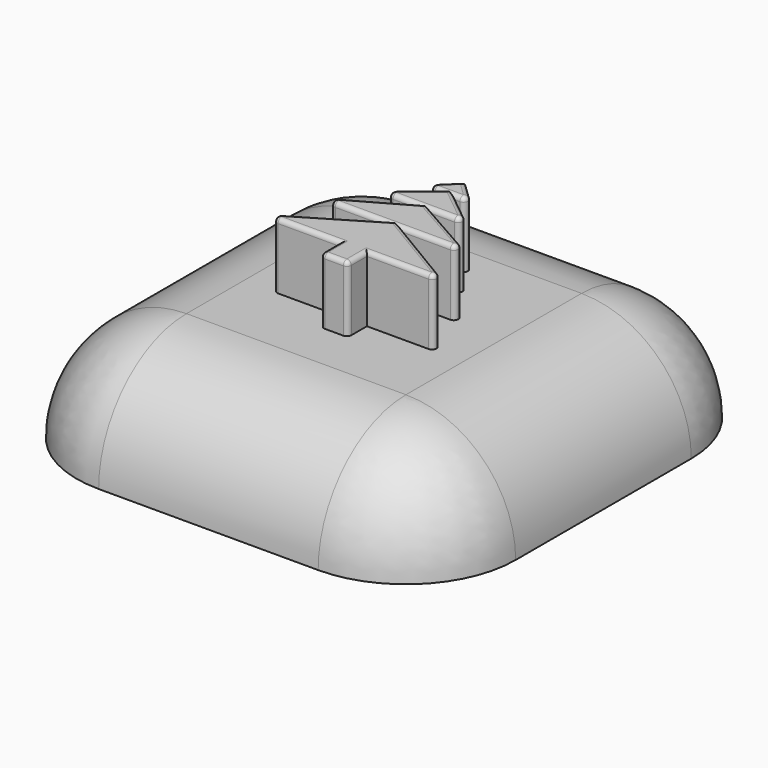
from build123d import *

# Parameters (mm, degrees)
F0_W          = 20
F0_H          = 20
F1_DEPTH      = 5
F2_R          = 4.99999
F3_T3_ANGLE   = 90
F3_T6_ANGLE   = 90
F3_T9_ANGLE   = 90
F3_T12_ANGLE  = 90
F3_T15_DEPTH  = 5
F3_T18_DEPTH  = 5
F3_T21_DEPTH  = 5
F3_T24_DEPTH  = 5
F5_DEPTH      = 3
F6_T1_DEPTH   = 4.0297756549
F6_T3_DEPTH   = 4.0297756549
F6_T5_DEPTH   = 2.2378753163
F6_T7_DEPTH   = 1.5910214623
F6_T9_DEPTH   = 2.4816952517
F6_T11_DEPTH  = 2.4816952517
F6_T16_DEPTH  = 2.7007100396
F6_T21_DEPTH  = 1.7701328723
F6_T26_DEPTH  = 1.7701328723
F6_T31_DEPTH  = 2.7007100396
F6_T36_DEPTH  = 3.9842649237
F6_T41_DEPTH  = 3.9842649237
F6_T46_DEPTH  = 5.3750440238
F6_T51_DEPTH  = 5.3750440238
F6_T56_DEPTH  = 4.5781609342
F6_T61_DEPTH  = 4.5781609342
F6_T66_DEPTH  = 3.1449194872
F6_T71_DEPTH  = 3.1449194872
F6_T77_DEPTH  = 2.7007100396
F6_T81_DEPTH  = 4.5781609342
F6_T88_DEPTH  = 1.7701328723
F6_T92_DEPTH  = 3.1449194872
F6_T99_DEPTH  = 3.1449194872
F6_T103_DEPTH = 1.7701328723
F6_T110_DEPTH = 2.7007100396
F6_T114_DEPTH = 4.5781609342
F6_T121_DEPTH = 5.3750440238
F6_T125_DEPTH = 3.9842649237
F6_T132_DEPTH = 3.9842649237
F6_T136_DEPTH = 5.3750440238
F6_T143_DEPTH = 4.5297756549
F6_T147_DEPTH = 2.0910214623
F6_T154_DEPTH = 2.0910214623
F6_T158_DEPTH = 4.5297756549
F7_T1_DEPTH   = 2.8
F7_T6_DEPTH   = 0.2
F7_T12_DEPTH  = 0.2
F7_T18_DEPTH  = 0.2
F7_T24_DEPTH  = 0.2
F7_S29_W      = 0.2
F7_S29_H      = 0.2
F7_T30_DEPTH  = 0.2
F7_S35_W      = 0.2
F7_S35_H      = 0.2
F7_T36_DEPTH  = 0.2
F7_T42_DEPTH  = 0.2
F7_T48_DEPTH  = 0.2
F7_T54_DEPTH  = 0.2
F7_T60_DEPTH  = 0.2


# Not quite as in the source:
# - a fillet or chamfer that OpenCascade refuses, or shapes differently, is made with other operations: its cross-section is extruded or revolved along the edge and cut away or added
# - a fillet or chamfer is up to 0.001 mm smaller than in the source, because OpenCascade refuses the exact size


with BuildPart() as f1:
    # F0 (on Top) → F1 (new body)
    with BuildSketch(Plane.XY):
        Rectangle(F0_W, F0_H)
    extrude(amount=-F1_DEPTH)

    # F2 (radius 5 in the source; OpenCascade refuses exactly that, so slightly less here)
    f2_edges = [f1.edges().sort_by_distance(p)[0] for p in [
        (0, 10, 0),
        (-10, 0, 0),
        (0, -10, 0),
        (10, 0, 0),
    ]]
    fillet(f2_edges, radius=F2_R)

    # F3: fillet of radius 5 on 5 edges, made by hand


with BuildPart() as f3_tool1:
    # F3_s2 → F3_t3 (revolve)
    with BuildSketch(Plane.YZ.offset(-5)):
        with BuildLine():
            ThreePointArc((5.00001, 0), (8.5355368349, -1.4644631651), (10, -4.99999))
            Line((10, -4.99999), (10, 0))
            Line((10, 0), (5.00001, 0))
        make_face()
    revolve(axis=Axis((-5, 5, 0), (0, 0, 1)), revolution_arc=F3_T3_ANGLE)


with BuildPart() as f3_tool4:
    # F3_s5 → F3_t6 (revolve)
    with BuildSketch(Plane.XZ.offset(-5)):
        with BuildLine():
            ThreePointArc((5.00001, 0), (8.5355368349, -1.4644631651), (10, -4.99999))
            Line((10, -4.99999), (10, 0))
            Line((10, 0), (5.00001, 0))
        make_face()
    revolve(axis=Axis((5, 5, 0), (0, 0, 1)), revolution_arc=F3_T6_ANGLE)


with BuildPart() as f3_tool7:
    # F3_s8 → F3_t9 (revolve)
    with BuildSketch(Plane.YZ.offset(5)):
        with BuildLine():
            ThreePointArc((-5.00001, 0), (-8.5355368349, -1.4644631651), (-10, -4.99999))
            Line((-10, -4.99999), (-10, 0))
            Line((-10, 0), (-5.00001, 0))
        make_face()
    revolve(axis=Axis((5, -5, 0), (0, 0, 1)), revolution_arc=F3_T9_ANGLE)


with BuildPart() as f3_tool10:
    # F3_s11 → F3_t12 (revolve)
    with BuildSketch(Plane.XZ.offset(5)):
        with BuildLine():
            ThreePointArc((-5.00001, 0), (-8.5355368349, -1.4644631651), (-10, -4.99999))
            Line((-10, -4.99999), (-10, 0))
            Line((-10, 0), (-5.00001, 0))
        make_face()
    revolve(axis=Axis((-5, -5, 0), (0, 0, 1)), revolution_arc=F3_T12_ANGLE)


with BuildPart() as f3_tool13:
    # F3_s14 → F3_t15 (new body)
    with BuildSketch(Plane.XY):
        with BuildLine():
            ThreePointArc((-5, -10), (-8.5355339059, -8.5355339059), (-10, -5))
            Line((-10, -5), (-10.1, -5))
            Line((-10.1, -5), (-10.1, -10.1))
            Line((-10.1, -10.1), (-5, -10.1))
            Line((-5, -10.1), (-5, -10))
        make_face()
    extrude(amount=-F3_T15_DEPTH)


with BuildPart() as f3_tool16:
    # F3_s17 → F3_t18 (new body)
    with BuildSketch(Plane.XY):
        with BuildLine():
            ThreePointArc((5, -10), (8.5355339059, -8.5355339059), (10, -5))
            Line((10, -5), (10.1, -5))
            Line((10.1, -5), (10.1, -10.1))
            Line((10.1, -10.1), (5, -10.1))
            Line((5, -10.1), (5, -10))
        make_face()
    extrude(amount=-F3_T18_DEPTH)


with BuildPart() as f3_tool19:
    # F3_s20 → F3_t21 (new body)
    with BuildSketch(Plane.XY):
        with BuildLine():
            ThreePointArc((10, 5), (8.5355339059, 8.5355339059), (5, 10))
            Line((5, 10), (5, 10.1))
            Line((5, 10.1), (10.1, 10.1))
            Line((10.1, 10.1), (10.1, 5))
            Line((10.1, 5), (10, 5))
        make_face()
    extrude(amount=-F3_T21_DEPTH)


with BuildPart() as f3_tool22:
    # F3_s23 → F3_t24 (new body)
    with BuildSketch(Plane.XY):
        with BuildLine():
            ThreePointArc((-10, 5), (-8.5355339059, 8.5355339059), (-5, 10))
            Line((-5, 10), (-5, 10.1))
            Line((-5, 10.1), (-10.1, 10.1))
            Line((-10.1, 10.1), (-10.1, 5))
            Line((-10.1, 5), (-10, 5))
        make_face()
    extrude(amount=-F3_T24_DEPTH)


with BuildPart() as f1_1:
    add(f1.part)

    # F3_t25: cut F3_tool1, F3_tool4, F3_tool7, F3_tool10, F3_tool13, F3_tool16, F3_tool19, F3_tool22
    add([f3_tool1.part, f3_tool4.part, f3_tool7.part, f3_tool10.part, f3_tool13.part, f3_tool16.part, f3_tool19.part, f3_tool22.part], mode=Mode.SUBTRACT)

    # F4 (on face) → F5 (join)
    with BuildSketch(Plane.XY):
        Polygon((1.0681818239, 3.6131960806), (0, 4.6400399879), (-1.0681818239, 3.6131960806), (-0.2980489517, 3.6131960806), (-1.9666701555, 2.2654635832), (-0.2659601159, 2.2654635832), (-3.3785805572, 0.5005755811), (-0.3943156335, 0.5005755811), (-4.148713313, -1.7456453061), (-0.6189376581, -1.7456453061), (-0.6189376581, -2.8366667684), (0, -2.8366667684), (0.6189376581, -2.8366667684), (0.6189376581, -1.7456453061), (4.148713313, -1.7456453061), (0.3943156335, 0.5005755811), (3.3785805572, 0.5005755811), (0.2659601159, 2.2654635832), (1.9666701555, 2.2654635832), (0.2980489517, 3.6131960806), align=None)
    extrude(amount=F5_DEPTH)

    # F6: fillet of radius 0.2 on 19 edges, made by hand

    # F6_s2 → F6_t1 (cut)
    with BuildSketch(Plane.YZ.offset(-4.648713313)):
        with BuildLine():
            ThreePointArc((-1.7456453061, 2.8), (-1.6870666623, 2.9414213562), (-1.5456453061, 3))
            Line((-1.5456453061, 3), (-1.7456453061, 3))
            Line((-1.7456453061, 3), (-1.7456453061, 2.8))
        make_face()
    extrude(amount=F6_T1_DEPTH, mode=Mode.SUBTRACT)

    # F6_s4 → F6_t3 (cut)
    with BuildSketch(Plane.YZ.offset(0.6189376581)):
        with BuildLine():
            ThreePointArc((-1.7456453061, 2.8), (-1.6870666623, 2.9414213562), (-1.5456453061, 3))
            Line((-1.5456453061, 3), (-1.7456453061, 3))
            Line((-1.7456453061, 3), (-1.7456453061, 2.8))
        make_face()
    extrude(amount=F6_T3_DEPTH, mode=Mode.SUBTRACT)

    # F6_s6 → F6_t5 (cut)
    with BuildSketch(Plane.YZ.offset(-1.1189376581)):
        with BuildLine():
            ThreePointArc((-2.8366667684, 2.8), (-2.7780881247, 2.9414213562), (-2.6366667684, 3))
            Line((-2.6366667684, 3), (-2.8366667684, 3))
            Line((-2.8366667684, 3), (-2.8366667684, 2.8))
        make_face()
    extrude(amount=F6_T5_DEPTH, mode=Mode.SUBTRACT)

    # F6_s8 → F6_t7 (cut)
    with BuildSketch(Plane.XZ.offset(1.7456453061)):
        with BuildLine():
            ThreePointArc((-0.6189376581, 2.8), (-0.5603590144, 2.9414213562), (-0.4189376581, 3))
            Line((-0.4189376581, 3), (-0.6189376581, 3))
            Line((-0.6189376581, 3), (-0.6189376581, 2.8))
        make_face()
        with BuildLine():
            ThreePointArc((0.6189376581, 2.8), (0.5603590144, 2.9414213562), (0.4189376581, 3))
            Line((0.4189376581, 3), (0.6189376581, 3))
            Line((0.6189376581, 3), (0.6189376581, 2.8))
        make_face()
    extrude(amount=F6_T7_DEPTH, mode=Mode.SUBTRACT)

    # F6_s10 → F6_t9 (cut)
    with BuildSketch(Plane(origin=(-0.8895730107, 0.8551471348, 0), x_dir=(0, 0, 1), z_dir=(-0.7209187063, 0.6930196382, 0))):
        with BuildLine():
            ThreePointArc((2.8, 3.345091625), (2.9414213562, 3.2865129813), (3, 3.145091625))
            Line((3, 3.145091625), (3, 3.345091625))
            Line((3, 3.345091625), (2.8, 3.345091625))
        make_face()
    extrude(amount=F6_T9_DEPTH, mode=Mode.SUBTRACT)

    # F6_s12 → F6_t11 (cut)
    with BuildSketch(Plane(origin=(2.6786735409, 2.5750106803, 0), x_dir=(0, 0, 1), z_dir=(-0.7209187063, -0.6930196382, 0))):
        with BuildLine():
            ThreePointArc((2.8, 3.345091625), (2.9414213562, 3.2865129813), (3, 3.145091625))
            Line((3, 3.145091625), (3, 3.345091625))
            Line((3, 3.345091625), (2.8, 3.345091625))
        make_face()
    extrude(amount=F6_T11_DEPTH, mode=Mode.SUBTRACT)


with BuildPart() as f6_tool14:
    # F6_s15 → F6_t16 (new body)
    with BuildSketch(Plane.YZ.offset(-2.4666701555)):
        with BuildLine():
            ThreePointArc((2.2654635832, 2.8), (2.3240422269, 2.9414213562), (2.4654635832, 3))
            Line((2.4654635832, 3), (2.2654635832, 3))
            Line((2.2654635832, 3), (2.2654635832, 2.8))
        make_face()
    extrude(amount=F6_T16_DEPTH)

    split(bisect_by=Plane(origin=(-1.036736214, 1.828425559, 0), x_dir=(0, 0, 1), z_dir=(-0.493238855, 0.8698939199, 0)), keep=Keep.TOP)


with BuildPart() as f1_2:
    add(f1_1.part)

    # F6_t13: cut F6_tool14
    add(f6_tool14.part, mode=Mode.SUBTRACT)


with BuildPart() as f6_tool19:
    # F6_s20 → F6_t21 (new body)
    with BuildSketch(Plane.YZ.offset(-1.5681818239)):
        with BuildLine():
            ThreePointArc((3.6131960806, 2.8), (3.6717747243, 2.9414213562), (3.8131960806, 3))
            Line((3.8131960806, 3), (3.6131960806, 3))
            Line((3.6131960806, 3), (3.6131960806, 2.8))
        make_face()
    extrude(amount=F6_T21_DEPTH)

    split(bisect_by=Plane(origin=(-1.8838358478, 2.3323682157, 0), x_dir=(0, 0, 1), z_dir=(-0.6283371033, 0.7779411833, 0)), keep=Keep.TOP)


with BuildPart() as f1_3:
    add(f1_2.part)

    # F6_t18: cut F6_tool19
    add(f6_tool19.part, mode=Mode.SUBTRACT)


with BuildPart() as f6_tool24:
    # F6_s25 → F6_t26 (new body)
    with BuildSketch(Plane.YZ.offset(-0.2019510483)):
        with BuildLine():
            ThreePointArc((3.6131960806, 2.8), (3.6717747243, 2.9414213562), (3.8131960806, 3))
            Line((3.8131960806, 3), (3.6131960806, 3))
            Line((3.6131960806, 3), (3.6131960806, 2.8))
        make_face()
    extrude(amount=F6_T26_DEPTH)

    split(bisect_by=Plane(origin=(1.8838358478, 2.3323682157, 0), x_dir=(0, 0, 1), z_dir=(0.6283371033, 0.7779411833, 0)), keep=Keep.TOP)


with BuildPart() as f1_4:
    add(f1_3.part)

    # F6_t23: cut F6_tool24
    add(f6_tool24.part, mode=Mode.SUBTRACT)


with BuildPart() as f6_tool29:
    # F6_s30 → F6_t31 (new body)
    with BuildSketch(Plane.YZ.offset(-0.2340398841)):
        with BuildLine():
            ThreePointArc((2.2654635832, 2.8), (2.3240422269, 2.9414213562), (2.4654635832, 3))
            Line((2.4654635832, 3), (2.2654635832, 3))
            Line((2.2654635832, 3), (2.2654635832, 2.8))
        make_face()
    extrude(amount=F6_T31_DEPTH)

    split(bisect_by=Plane(origin=(1.036736214, 1.828425559, 0), x_dir=(0, 0, 1), z_dir=(0.493238855, 0.8698939199, 0)), keep=Keep.TOP)


with BuildPart() as f1_5:
    add(f1_4.part)

    # F6_t28: cut F6_tool29
    add(f6_tool29.part, mode=Mode.SUBTRACT)


with BuildPart() as f6_tool34:
    # F6_s35 → F6_t36 (new body)
    with BuildSketch(Plane.YZ.offset(-0.1056843665)):
        with BuildLine():
            ThreePointArc((0.5005755811, 2.8), (0.5591542249, 2.9414213562), (0.7005755811, 3))
            Line((0.7005755811, 3), (0.5005755811, 3))
            Line((0.5005755811, 3), (0.5005755811, 2.8))
        make_face()
    extrude(amount=F6_T36_DEPTH)

    split(bisect_by=Plane(origin=(0.3244854875, 0.5423543019, 0), x_dir=(0, 0, 1), z_dir=(0.5134167508, 0.8581394059, 0)), keep=Keep.TOP)


with BuildPart() as f1_6:
    add(f1_5.part)

    # F6_t33: cut F6_tool34
    add(f6_tool34.part, mode=Mode.SUBTRACT)


with BuildPart() as f6_tool39:
    # F6_s40 → F6_t41 (new body)
    with BuildSketch(Plane.YZ.offset(-3.8785805572)):
        with BuildLine():
            ThreePointArc((0.5005755811, 2.8), (0.5591542249, 2.9414213562), (0.7005755811, 3))
            Line((0.7005755811, 3), (0.5005755811, 3))
            Line((0.5005755811, 3), (0.5005755811, 2.8))
        make_face()
    extrude(amount=F6_T41_DEPTH)

    split(bisect_by=Plane(origin=(-0.3244854875, 0.5423543019, 0), x_dir=(0, 0, 1), z_dir=(-0.5134167508, 0.8581394059, 0)), keep=Keep.TOP)


with BuildPart() as f1_7:
    add(f1_6.part)

    # F6_t38: cut F6_tool39
    add(f6_tool39.part, mode=Mode.SUBTRACT)


with BuildPart() as f6_tool44:
    # F6_s45 → F6_t46 (new body)
    with BuildSketch(Plane(origin=(4.2532975285, -2.5447079834, 0), x_dir=(0, 0, 1), z_dir=(-0.8581394059, 0.5134167508, 0))):
        with BuildLine():
            ThreePointArc((2.8, 0.6320118831), (2.9414213562, 0.5734332393), (3, 0.4320118831))
            Line((3, 0.4320118831), (3, 0.6320118831))
            Line((3, 0.6320118831), (2.8, 0.6320118831))
        make_face()
    extrude(amount=F6_T46_DEPTH)

    split(bisect_by=Plane.XZ.offset(-0.5005755811), keep=Keep.TOP)


with BuildPart() as f1_8:
    add(f1_7.part)

    # F6_t43: cut F6_tool44
    add(f6_tool44.part, mode=Mode.SUBTRACT)


with BuildPart() as f6_tool49:
    # F6_s50 → F6_t51 (new body)
    with BuildSketch(Plane(origin=(0.359239557, 0.2149296546, 0), x_dir=(0, 0, 1), z_dir=(-0.8581394059, -0.5134167508, 0))):
        with BuildLine():
            ThreePointArc((2.8, 0.6320118831), (2.9414213562, 0.5734332393), (3, 0.4320118831))
            Line((3, 0.4320118831), (3, 0.6320118831))
            Line((3, 0.6320118831), (2.8, 0.6320118831))
        make_face()
    extrude(amount=F6_T51_DEPTH)

    split(bisect_by=Plane.XZ.offset(-0.5005755811), keep=Keep.TOP)


with BuildPart() as f1_9:
    add(f1_8.part)

    # F6_t48: cut F6_tool49
    add(f6_tool49.part, mode=Mode.SUBTRACT)


with BuildPart() as f6_tool54:
    # F6_s55 → F6_t56 (new body)
    with BuildSketch(Plane(origin=(1.205723058, 0.6836574517, 0), x_dir=(0, 0, 1), z_dir=(-0.8698939199, -0.493238855, 0))):
        with BuildLine():
            ThreePointArc((2.8, 2.1018948599), (2.9414213562, 2.0433162161), (3, 1.9018948599))
            Line((3, 1.9018948599), (3, 2.1018948599))
            Line((3, 2.1018948599), (2.8, 2.1018948599))
        make_face()
    extrude(amount=F6_T56_DEPTH)

    split(bisect_by=Plane.XZ.offset(-2.2654635832), keep=Keep.TOP)


with BuildPart() as f1_10:
    add(f1_9.part)

    # F6_t53: cut F6_tool54
    add(f6_tool54.part, mode=Mode.SUBTRACT)


with BuildPart() as f6_tool59:
    # F6_s60 → F6_t61 (new body)
    with BuildSketch(Plane(origin=(2.7767913032, -1.5744694054, 0), x_dir=(0, 0, 1), z_dir=(-0.8698939199, 0.493238855, 0))):
        with BuildLine():
            ThreePointArc((2.8, 2.1018948599), (2.9414213562, 2.0433162161), (3, 1.9018948599))
            Line((3, 1.9018948599), (3, 2.1018948599))
            Line((3, 2.1018948599), (2.8, 2.1018948599))
        make_face()
    extrude(amount=F6_T61_DEPTH)

    split(bisect_by=Plane.XZ.offset(-2.2654635832), keep=Keep.TOP)


with BuildPart() as f1_11:
    add(f1_10.part)

    # F6_t58: cut F6_tool59
    add(f6_tool59.part, mode=Mode.SUBTRACT)


with BuildPart() as f6_tool64:
    # F6_s65 → F6_t66 (new body)
    with BuildSketch(Plane(origin=(0.4718048994, -0.3810731842, 0), x_dir=(0, 0, 1), z_dir=(-0.7779411833, 0.6283371033, 0))):
        with BuildLine():
            ThreePointArc((2.8, 2.9981292492), (2.9414213562, 2.9395506054), (3, 2.7981292492))
            Line((3, 2.7981292492), (3, 2.9981292492))
            Line((3, 2.9981292492), (2.8, 2.9981292492))
        make_face()
    extrude(amount=F6_T66_DEPTH)

    split(bisect_by=Plane.XZ.offset(-3.6131960806), keep=Keep.TOP)


with BuildPart() as f1_12:
    add(f1_11.part)

    # F6_t63: cut F6_tool64
    add(f6_tool64.part, mode=Mode.SUBTRACT)


with BuildPart() as f6_tool69:
    # F6_s70 → F6_t71 (new body)
    with BuildSketch(Plane(origin=(1.9747574877, 1.5949964165, 0), x_dir=(0, 0, 1), z_dir=(-0.7779411833, -0.6283371033, 0))):
        with BuildLine():
            ThreePointArc((2.8, 2.9981292492), (2.9414213562, 2.9395506054), (3, 2.7981292492))
            Line((3, 2.7981292492), (3, 2.9981292492))
            Line((3, 2.9981292492), (2.8, 2.9981292492))
        make_face()
    extrude(amount=F6_T71_DEPTH)

    split(bisect_by=Plane.XZ.offset(-3.6131960806), keep=Keep.TOP)


with BuildPart() as f1_13:
    add(f1_12.part)

    # F6_t68: cut F6_tool69
    add(f6_tool69.part, mode=Mode.SUBTRACT)


with BuildPart() as f6_tool75:
    # F6_s76 → F6_t77 (new body)
    with BuildSketch(Plane.YZ.offset(-2.4666701555)):
        with BuildLine():
            ThreePointArc((2.2654635832, 2.8), (2.3240422269, 2.9414213562), (2.4654635832, 3))
            Line((2.4654635832, 3), (2.2654635832, 3))
            Line((2.2654635832, 3), (2.2654635832, 2.8))
        make_face()
    extrude(amount=F6_T77_DEPTH)

    split(bisect_by=Plane(origin=(-1.036736214, 1.828425559, 0), x_dir=(0, 0, 1), z_dir=(0.493238855, -0.8698939199, 0)), keep=Keep.TOP)


with BuildPart() as f6_tool79:
    # F6_s80 → F6_t81 (new body)
    with BuildSketch(Plane(origin=(1.205723058, 0.6836574517, 0), x_dir=(0, 0, 1), z_dir=(-0.8698939199, -0.493238855, 0))):
        with BuildLine():
            ThreePointArc((2.8, 2.1018948599), (2.9414213562, 2.0433162161), (3, 1.9018948599))
            Line((3, 1.9018948599), (3, 2.1018948599))
            Line((3, 2.1018948599), (2.8, 2.1018948599))
        make_face()
    extrude(amount=F6_T81_DEPTH)

    split(bisect_by=Plane.XZ.offset(-2.2654635832), keep=Keep.BOTTOM)


with BuildPart() as f6_tool75_1:
    add(f6_tool75.part)

    # F6_t83: intersect F6_tool79
    add(f6_tool79.part, mode=Mode.INTERSECT)


with BuildPart() as f1_14:
    add(f1_13.part)

    # F6_t73: cut F6_tool75
    add(f6_tool75_1.part, mode=Mode.SUBTRACT)


with BuildPart() as f6_tool86:
    # F6_s87 → F6_t88 (new body)
    with BuildSketch(Plane.YZ.offset(-1.5681818239)):
        with BuildLine():
            ThreePointArc((3.6131960806, 2.8), (3.6717747243, 2.9414213562), (3.8131960806, 3))
            Line((3.8131960806, 3), (3.6131960806, 3))
            Line((3.6131960806, 3), (3.6131960806, 2.8))
        make_face()
    extrude(amount=F6_T88_DEPTH)

    split(bisect_by=Plane(origin=(-1.8838358478, 2.3323682157, 0), x_dir=(0, 0, 1), z_dir=(0.6283371033, -0.7779411833, 0)), keep=Keep.TOP)


with BuildPart() as f6_tool90:
    # F6_s91 → F6_t92 (new body)
    with BuildSketch(Plane(origin=(1.9747574877, 1.5949964165, 0), x_dir=(0, 0, 1), z_dir=(-0.7779411833, -0.6283371033, 0))):
        with BuildLine():
            ThreePointArc((2.8, 2.9981292492), (2.9414213562, 2.9395506054), (3, 2.7981292492))
            Line((3, 2.7981292492), (3, 2.9981292492))
            Line((3, 2.9981292492), (2.8, 2.9981292492))
        make_face()
    extrude(amount=F6_T92_DEPTH)

    split(bisect_by=Plane.XZ.offset(-3.6131960806), keep=Keep.BOTTOM)


with BuildPart() as f6_tool86_1:
    add(f6_tool86.part)

    # F6_t94: intersect F6_tool90
    add(f6_tool90.part, mode=Mode.INTERSECT)


with BuildPart() as f1_15:
    add(f1_14.part)

    # F6_t84: cut F6_tool86
    add(f6_tool86_1.part, mode=Mode.SUBTRACT)


with BuildPart() as f6_tool97:
    # F6_s98 → F6_t99 (new body)
    with BuildSketch(Plane(origin=(0.4718048994, -0.3810731842, 0), x_dir=(0, 0, 1), z_dir=(-0.7779411833, 0.6283371033, 0))):
        with BuildLine():
            ThreePointArc((2.8, 2.9981292492), (2.9414213562, 2.9395506054), (3, 2.7981292492))
            Line((3, 2.7981292492), (3, 2.9981292492))
            Line((3, 2.9981292492), (2.8, 2.9981292492))
        make_face()
    extrude(amount=F6_T99_DEPTH)

    split(bisect_by=Plane.XZ.offset(-3.6131960806), keep=Keep.BOTTOM)


with BuildPart() as f6_tool101:
    # F6_s102 → F6_t103 (new body)
    with BuildSketch(Plane.YZ.offset(-0.2019510483)):
        with BuildLine():
            ThreePointArc((3.6131960806, 2.8), (3.6717747243, 2.9414213562), (3.8131960806, 3))
            Line((3.8131960806, 3), (3.6131960806, 3))
            Line((3.6131960806, 3), (3.6131960806, 2.8))
        make_face()
    extrude(amount=F6_T103_DEPTH)

    split(bisect_by=Plane(origin=(1.8838358478, 2.3323682157, 0), x_dir=(0, 0, 1), z_dir=(-0.6283371033, -0.7779411833, 0)), keep=Keep.TOP)


with BuildPart() as f6_tool97_1:
    add(f6_tool97.part)

    # F6_t105: intersect F6_tool101
    add(f6_tool101.part, mode=Mode.INTERSECT)


with BuildPart() as f1_16:
    add(f1_15.part)

    # F6_t95: cut F6_tool97
    add(f6_tool97_1.part, mode=Mode.SUBTRACT)


with BuildPart() as f6_tool108:
    # F6_s109 → F6_t110 (new body)
    with BuildSketch(Plane.YZ.offset(-0.2340398841)):
        with BuildLine():
            ThreePointArc((2.2654635832, 2.8), (2.3240422269, 2.9414213562), (2.4654635832, 3))
            Line((2.4654635832, 3), (2.2654635832, 3))
            Line((2.2654635832, 3), (2.2654635832, 2.8))
        make_face()
    extrude(amount=F6_T110_DEPTH)

    split(bisect_by=Plane(origin=(1.036736214, 1.828425559, 0), x_dir=(0, 0, 1), z_dir=(-0.493238855, -0.8698939199, 0)), keep=Keep.TOP)


with BuildPart() as f6_tool112:
    # F6_s113 → F6_t114 (new body)
    with BuildSketch(Plane(origin=(2.7767913032, -1.5744694054, 0), x_dir=(0, 0, 1), z_dir=(-0.8698939199, 0.493238855, 0))):
        with BuildLine():
            ThreePointArc((2.8, 2.1018948599), (2.9414213562, 2.0433162161), (3, 1.9018948599))
            Line((3, 1.9018948599), (3, 2.1018948599))
            Line((3, 2.1018948599), (2.8, 2.1018948599))
        make_face()
    extrude(amount=F6_T114_DEPTH)

    split(bisect_by=Plane.XZ.offset(-2.2654635832), keep=Keep.BOTTOM)


with BuildPart() as f6_tool108_1:
    add(f6_tool108.part)

    # F6_t116: intersect F6_tool112
    add(f6_tool112.part, mode=Mode.INTERSECT)


with BuildPart() as f1_17:
    add(f1_16.part)

    # F6_t106: cut F6_tool108
    add(f6_tool108_1.part, mode=Mode.SUBTRACT)


with BuildPart() as f6_tool119:
    # F6_s120 → F6_t121 (new body)
    with BuildSketch(Plane(origin=(4.2532975285, -2.5447079834, 0), x_dir=(0, 0, 1), z_dir=(-0.8581394059, 0.5134167508, 0))):
        with BuildLine():
            ThreePointArc((2.8, 0.6320118831), (2.9414213562, 0.5734332393), (3, 0.4320118831))
            Line((3, 0.4320118831), (3, 0.6320118831))
            Line((3, 0.6320118831), (2.8, 0.6320118831))
        make_face()
    extrude(amount=F6_T121_DEPTH)

    split(bisect_by=Plane.XZ.offset(-0.5005755811), keep=Keep.BOTTOM)


with BuildPart() as f6_tool123:
    # F6_s124 → F6_t125 (new body)
    with BuildSketch(Plane.YZ.offset(-0.1056843665)):
        with BuildLine():
            ThreePointArc((0.5005755811, 2.8), (0.5591542249, 2.9414213562), (0.7005755811, 3))
            Line((0.7005755811, 3), (0.5005755811, 3))
            Line((0.5005755811, 3), (0.5005755811, 2.8))
        make_face()
    extrude(amount=F6_T125_DEPTH)

    split(bisect_by=Plane(origin=(0.3244854875, 0.5423543019, 0), x_dir=(0, 0, 1), z_dir=(-0.5134167508, -0.8581394059, 0)), keep=Keep.TOP)


with BuildPart() as f6_tool119_1:
    add(f6_tool119.part)

    # F6_t127: intersect F6_tool123
    add(f6_tool123.part, mode=Mode.INTERSECT)


with BuildPart() as f1_18:
    add(f1_17.part)

    # F6_t117: cut F6_tool119
    add(f6_tool119_1.part, mode=Mode.SUBTRACT)


with BuildPart() as f6_tool130:
    # F6_s131 → F6_t132 (new body)
    with BuildSketch(Plane.YZ.offset(-3.8785805572)):
        with BuildLine():
            ThreePointArc((0.5005755811, 2.8), (0.5591542249, 2.9414213562), (0.7005755811, 3))
            Line((0.7005755811, 3), (0.5005755811, 3))
            Line((0.5005755811, 3), (0.5005755811, 2.8))
        make_face()
    extrude(amount=F6_T132_DEPTH)

    split(bisect_by=Plane(origin=(-0.3244854875, 0.5423543019, 0), x_dir=(0, 0, 1), z_dir=(0.5134167508, -0.8581394059, 0)), keep=Keep.TOP)


with BuildPart() as f6_tool134:
    # F6_s135 → F6_t136 (new body)
    with BuildSketch(Plane(origin=(0.359239557, 0.2149296546, 0), x_dir=(0, 0, 1), z_dir=(-0.8581394059, -0.5134167508, 0))):
        with BuildLine():
            ThreePointArc((2.8, 0.6320118831), (2.9414213562, 0.5734332393), (3, 0.4320118831))
            Line((3, 0.4320118831), (3, 0.6320118831))
            Line((3, 0.6320118831), (2.8, 0.6320118831))
        make_face()
    extrude(amount=F6_T136_DEPTH)

    split(bisect_by=Plane.XZ.offset(-0.5005755811), keep=Keep.BOTTOM)


with BuildPart() as f6_tool130_1:
    add(f6_tool130.part)

    # F6_t138: intersect F6_tool134
    add(f6_tool134.part, mode=Mode.INTERSECT)


with BuildPart() as f1_19:
    add(f1_18.part)

    # F6_t128: cut F6_tool130
    add(f6_tool130_1.part, mode=Mode.SUBTRACT)


with BuildPart() as f6_tool141:
    # F6_s142 → F6_t143 (new body)
    with BuildSketch(Plane.YZ.offset(-4.648713313)):
        with BuildLine():
            ThreePointArc((-1.7456453061, 2.8), (-1.6870666623, 2.9414213562), (-1.5456453061, 3))
            Line((-1.5456453061, 3), (-1.7456453061, 3))
            Line((-1.7456453061, 3), (-1.7456453061, 2.8))
        make_face()
    extrude(amount=F6_T143_DEPTH)

    split(bisect_by=Plane.YZ.offset(-0.6189376581), keep=Keep.TOP)


with BuildPart() as f6_tool145:
    # F6_s146 → F6_t147 (new body)
    with BuildSketch(Plane.XZ.offset(1.2456453061)):
        with BuildLine():
            ThreePointArc((-0.6189376581, 2.8), (-0.5603590144, 2.9414213562), (-0.4189376581, 3))
            Line((-0.4189376581, 3), (-0.6189376581, 3))
            Line((-0.6189376581, 3), (-0.6189376581, 2.8))
        make_face()
    extrude(amount=F6_T147_DEPTH)

    split(bisect_by=Plane.XZ.offset(1.7456453061), keep=Keep.BOTTOM)


with BuildPart() as f6_tool141_1:
    add(f6_tool141.part)

    # F6_t149: intersect F6_tool145
    add(f6_tool145.part, mode=Mode.INTERSECT)


with BuildPart() as f1_20:
    add(f1_19.part)

    # F6_t139: cut F6_tool141
    add(f6_tool141_1.part, mode=Mode.SUBTRACT)


with BuildPart() as f6_tool152:
    # F6_s153 → F6_t154 (new body)
    with BuildSketch(Plane.XZ.offset(3.3366667684)):
        with BuildLine():
            ThreePointArc((0.6189376581, 2.8), (0.5603590144, 2.9414213562), (0.4189376581, 3))
            Line((0.4189376581, 3), (0.6189376581, 3))
            Line((0.6189376581, 3), (0.6189376581, 2.8))
        make_face()
    extrude(amount=-F6_T154_DEPTH)

    split(bisect_by=Plane.XZ.offset(1.7456453061), keep=Keep.BOTTOM)


with BuildPart() as f6_tool156:
    # F6_s157 → F6_t158 (new body)
    with BuildSketch(Plane.YZ.offset(0.1189376581)):
        with BuildLine():
            ThreePointArc((-1.7456453061, 2.8), (-1.6870666623, 2.9414213562), (-1.5456453061, 3))
            Line((-1.5456453061, 3), (-1.7456453061, 3))
            Line((-1.7456453061, 3), (-1.7456453061, 2.8))
        make_face()
    extrude(amount=F6_T158_DEPTH)

    split(bisect_by=Plane.YZ.offset(0.6189376581), keep=Keep.BOTTOM)


with BuildPart() as f6_tool152_1:
    add(f6_tool152.part)

    # F6_t160: intersect F6_tool156
    add(f6_tool156.part, mode=Mode.INTERSECT)


with BuildPart() as f1_21:
    add(f1_20.part)

    # F6_t150: cut F6_tool152
    add(f6_tool152_1.part, mode=Mode.SUBTRACT)

    # F7: fillet of radius 0.2 on 10 edges, made by hand

    # F7_s2 → F7_t1 (cut)
    with BuildSketch(Plane.XY):
        with BuildLine():
            ThreePointArc((0.7101421902, 3.9573798218), (0.7570601592, 3.738485801), (0.5715382625, 3.6131960806))
            Line((0.5715382625, 3.6131960806), (1.0681818239, 3.6131960806))
            Line((1.0681818239, 3.6131960806), (0.7101421902, 3.9573798218))
        make_face()
        with BuildLine():
            ThreePointArc((1.5264180486, 2.6210518198), (1.589321102, 2.3988214318), (1.400750628, 2.2654635832))
            Line((1.400750628, 2.2654635832), (1.9666701555, 2.2654635832))
            Line((1.9666701555, 2.2654635832), (1.5264180486, 2.6210518198))
        make_face()
        with BuildLine():
            ThreePointArc((2.7190180205, 0.8745543651), (2.8137555602, 0.6495645862), (2.6203702495, 0.5005755811))
            Line((2.6203702495, 0.5005755811), (3.3785805572, 0.5005755811))
            Line((3.3785805572, 0.5005755811), (2.7190180205, 0.8745543651))
        make_face()
        with BuildLine():
            ThreePointArc((3.5275638692, -1.3740174249), (3.6176570428, -1.598910791), (3.4248805191, -1.7456453061))
            Line((3.4248805191, -1.7456453061), (4.148713313, -1.7456453061))
            Line((4.148713313, -1.7456453061), (3.5275638692, -1.3740174249))
        make_face()
        with BuildLine():
            ThreePointArc((0.6189376581, -2.6366667684), (0.5603590144, -2.7780881247), (0.4189376581, -2.8366667684))
            Line((0.4189376581, -2.8366667684), (0.6189376581, -2.8366667684))
            Line((0.6189376581, -2.8366667684), (0.6189376581, -2.6366667684))
        make_face()
        with BuildLine():
            ThreePointArc((-0.4189376581, -2.8366667684), (-0.5603590144, -2.7780881247), (-0.6189376581, -2.6366667684))
            Line((-0.6189376581, -2.6366667684), (-0.6189376581, -2.8366667684))
            Line((-0.6189376581, -2.8366667684), (-0.4189376581, -2.8366667684))
        make_face()
        with BuildLine():
            ThreePointArc((-2.6203702495, 0.5005755811), (-2.8137555602, 0.6495645862), (-2.7190180205, 0.8745543651))
            Line((-2.7190180205, 0.8745543651), (-3.3785805572, 0.5005755811))
            Line((-3.3785805572, 0.5005755811), (-2.6203702495, 0.5005755811))
        make_face()
        with BuildLine():
            ThreePointArc((-1.400750628, 2.2654635832), (-1.589321102, 2.3988214318), (-1.5264180486, 2.6210518198))
            Line((-1.5264180486, 2.6210518198), (-1.9666701555, 2.2654635832))
            Line((-1.9666701555, 2.2654635832), (-1.400750628, 2.2654635832))
        make_face()
        with BuildLine():
            ThreePointArc((-0.5715382625, 3.6131960806), (-0.7570601592, 3.738485801), (-0.7101421902, 3.9573798218))
            Line((-0.7101421902, 3.9573798218), (-1.0681818239, 3.6131960806))
            Line((-1.0681818239, 3.6131960806), (-0.5715382625, 3.6131960806))
        make_face()
        with BuildLine():
            ThreePointArc((-3.4248805191, -1.7456453061), (-3.6176570428, -1.598910791), (-3.5275638692, -1.3740174249))
            Line((-3.5275638692, -1.3740174249), (-4.148713313, -1.7456453061))
            Line((-4.148713313, -1.7456453061), (-3.4248805191, -1.7456453061))
        make_face()
    extrude(amount=F7_T1_DEPTH, mode=Mode.SUBTRACT)


with BuildPart() as f7_tool4:
    # F7_s5 → F7_t6 (new body)
    with BuildSketch(Plane.XY.offset(2.8)):
        Polygon((-3.4248805191, -1.5456453061), (-3.4248805191, -1.7456453061), (-4.148713313, -1.7456453061), (-3.5275638692, -1.3740174249), align=None)
    extrude(amount=F7_T6_DEPTH)

    # F7_s7 → F7_t8 (revolve, cut)
    with BuildSketch(Plane(origin=(-3.4248805191, -1.5456453061, 2.8), x_dir=(0.9638826189, 0.2663274245, 0), z_dir=(0.2663274245, -0.9638826189, 0))):
        with BuildLine():
            ThreePointArc((0, -0.2), (0.2, 0), (0, 0.2))
            Line((0, 0.2), (0, -0.2))
        make_face()
    revolve(axis=Axis((-3.4248805191, -1.5456453061, 2.8), (0, 0, 1)), mode=Mode.SUBTRACT)


with BuildPart() as f1_22:
    add(f1_21.part)

    # F7_t3: cut F7_tool4
    add(f7_tool4.part, mode=Mode.SUBTRACT)


with BuildPart() as f7_tool10:
    # F7_s11 → F7_t12 (new body)
    with BuildSketch(Plane.XY.offset(2.8)):
        Polygon((-0.5715382625, 3.8131960806), (-0.5715382625, 3.6131960806), (-1.0681818239, 3.6131960806), (-0.7101421902, 3.9573798218), align=None)
    extrude(amount=F7_T12_DEPTH)

    # F7_s13 → F7_t14 (revolve, cut)
    with BuildSketch(Plane(origin=(-0.5715382625, 3.8131960806, 2.8), x_dir=(0.9276094831, 0.3735513979, 0), z_dir=(0.3735513979, -0.9276094831, 0))):
        with BuildLine():
            ThreePointArc((0, -0.2), (0.2, 0), (0, 0.2))
            Line((0, 0.2), (0, -0.2))
        make_face()
    revolve(axis=Axis((-0.5715382625, 3.8131960806, 2.8), (0, 0, 1)), mode=Mode.SUBTRACT)


with BuildPart() as f1_23:
    add(f1_22.part)

    # F7_t9: cut F7_tool10
    add(f7_tool10.part, mode=Mode.SUBTRACT)


with BuildPart() as f7_tool16:
    # F7_s17 → F7_t18 (new body)
    with BuildSketch(Plane.XY.offset(2.8)):
        Polygon((-1.400750628, 2.4654635832), (-1.400750628, 2.2654635832), (-1.9666701555, 2.2654635832), (-1.5264180486, 2.6210518198), align=None)
    extrude(amount=F7_T18_DEPTH)

    # F7_s19 → F7_t20 (revolve, cut)
    with BuildSketch(Plane(origin=(-1.400750628, 2.4654635832, 2.8), x_dir=(0.94285237, 0.3332107567, 0), z_dir=(0.3332107567, -0.94285237, 0))):
        with BuildLine():
            ThreePointArc((0, -0.2), (0.2, 0), (0, 0.2))
            Line((0, 0.2), (0, -0.2))
        make_face()
    revolve(axis=Axis((-1.400750628, 2.4654635832, 2.8), (0, 0, 1)), mode=Mode.SUBTRACT)


with BuildPart() as f1_24:
    add(f1_23.part)

    # F7_t15: cut F7_tool16
    add(f7_tool16.part, mode=Mode.SUBTRACT)


with BuildPart() as f7_tool22:
    # F7_s23 → F7_t24 (new body)
    with BuildSketch(Plane.XY.offset(2.8)):
        Polygon((-2.6203702495, 0.7005755811), (-2.6203702495, 0.5005755811), (-3.3785805572, 0.5005755811), (-2.7190180205, 0.8745543651), align=None)
    extrude(amount=F7_T24_DEPTH)

    # F7_s25 → F7_t26 (revolve, cut)
    with BuildSketch(Plane(origin=(-2.6203702495, 0.7005755811, 2.8), x_dir=(0.9669265536, 0.2550549745, 0), z_dir=(0.2550549745, -0.9669265536, 0))):
        with BuildLine():
            ThreePointArc((0, -0.2), (0.2, 0), (0, 0.2))
            Line((0, 0.2), (0, -0.2))
        make_face()
    revolve(axis=Axis((-2.6203702495, 0.7005755811, 2.8), (0, 0, 1)), mode=Mode.SUBTRACT)


with BuildPart() as f1_25:
    add(f1_24.part)

    # F7_t21: cut F7_tool22
    add(f7_tool22.part, mode=Mode.SUBTRACT)


with BuildPart() as f7_tool28:
    # F7_s29 → F7_t30 (new body)
    with BuildSketch(Plane.XZ.offset(2.6366667684)):
        with Locations((-0.5189376581, 2.9)):
            Rectangle(F7_S29_W, F7_S29_H)
    extrude(amount=F7_T30_DEPTH)

    # F7_s31 → F7_t32 (revolve, cut)
    with BuildSketch(Plane(origin=(-0.4189376581, -2.6366667684, 2.8), x_dir=(0.7071067812, 0, -0.7071067812), z_dir=(-0.7071067812, 0, -0.7071067812))):
        with BuildLine():
            ThreePointArc((0, -0.2), (0.2, 0), (0, 0.2))
            Line((0, 0.2), (0, -0.2))
        make_face()
    revolve(axis=Axis((-0.4189376581, -2.6366667684, 2.8), (0, -1, 0)), mode=Mode.SUBTRACT)


with BuildPart() as f1_26:
    add(f1_25.part)

    # F7_t27: cut F7_tool28
    add(f7_tool28.part, mode=Mode.SUBTRACT)


with BuildPart() as f7_tool34:
    # F7_s35 → F7_t36 (new body)
    with BuildSketch(Plane.YZ.offset(0.4189376581)):
        with Locations((-2.7366667684, 2.9)):
            Rectangle(F7_S35_W, F7_S35_H)
    extrude(amount=F7_T36_DEPTH)

    # F7_s37 → F7_t38 (revolve, cut)
    with BuildSketch(Plane(origin=(0.4189376581, -2.6366667684, 2.8), x_dir=(0, 0.7071067812, -0.7071067812), z_dir=(0, -0.7071067812, -0.7071067812))):
        with BuildLine():
            ThreePointArc((0, -0.2), (0.2, 0), (0, 0.2))
            Line((0, 0.2), (0, -0.2))
        make_face()
    revolve(axis=Axis((0.4189376581, -2.6366667684, 2.8), (1, 0, 0)), mode=Mode.SUBTRACT)


with BuildPart() as f1_27:
    add(f1_26.part)

    # F7_t33: cut F7_tool34
    add(f7_tool34.part, mode=Mode.SUBTRACT)


with BuildPart() as f7_tool40:
    # F7_s41 → F7_t42 (new body)
    with BuildSketch(Plane.XY.offset(2.8)):
        Polygon((3.4248805191, -1.5456453061), (3.5275638692, -1.3740174249), (4.148713313, -1.7456453061), (3.4248805191, -1.7456453061), align=None)
    extrude(amount=F7_T42_DEPTH)

    # F7_s43 → F7_t44 (revolve, cut)
    with BuildSketch(Plane(origin=(3.4248805191, -1.5456453061, 2.8), x_dir=(-0.9638826189, 0.2663274245, 0), z_dir=(0.2663274245, 0.9638826189, 0))):
        with BuildLine():
            ThreePointArc((0, -0.2), (0.2, 0), (0, 0.2))
            Line((0, 0.2), (0, -0.2))
        make_face()
    revolve(axis=Axis((3.4248805191, -1.5456453061, 2.8), (0, 0, 1)), mode=Mode.SUBTRACT)


with BuildPart() as f1_28:
    add(f1_27.part)

    # F7_t39: cut F7_tool40
    add(f7_tool40.part, mode=Mode.SUBTRACT)


with BuildPart() as f7_tool46:
    # F7_s47 → F7_t48 (new body)
    with BuildSketch(Plane.XY.offset(2.8)):
        Polygon((2.6203702495, 0.7005755811), (2.7190180205, 0.8745543651), (3.3785805572, 0.5005755811), (2.6203702495, 0.5005755811), align=None)
    extrude(amount=F7_T48_DEPTH)

    # F7_s49 → F7_t50 (revolve, cut)
    with BuildSketch(Plane(origin=(2.6203702495, 0.7005755811, 2.8), x_dir=(-0.9669265536, 0.2550549745, 0), z_dir=(0.2550549745, 0.9669265536, 0))):
        with BuildLine():
            ThreePointArc((0, -0.2), (0.2, 0), (0, 0.2))
            Line((0, 0.2), (0, -0.2))
        make_face()
    revolve(axis=Axis((2.6203702495, 0.7005755811, 2.8), (0, 0, 1)), mode=Mode.SUBTRACT)


with BuildPart() as f1_29:
    add(f1_28.part)

    # F7_t45: cut F7_tool46
    add(f7_tool46.part, mode=Mode.SUBTRACT)


with BuildPart() as f7_tool52:
    # F7_s53 → F7_t54 (new body)
    with BuildSketch(Plane.XY.offset(2.8)):
        Polygon((1.400750628, 2.4654635832), (1.5264180486, 2.6210518198), (1.9666701555, 2.2654635832), (1.400750628, 2.2654635832), align=None)
    extrude(amount=F7_T54_DEPTH)

    # F7_s55 → F7_t56 (revolve, cut)
    with BuildSketch(Plane(origin=(1.400750628, 2.4654635832, 2.8), x_dir=(-0.94285237, 0.3332107567, 0), z_dir=(0.3332107567, 0.94285237, 0))):
        with BuildLine():
            ThreePointArc((0, -0.2), (0.2, 0), (0, 0.2))
            Line((0, 0.2), (0, -0.2))
        make_face()
    revolve(axis=Axis((1.400750628, 2.4654635832, 2.8), (0, 0, 1)), mode=Mode.SUBTRACT)


with BuildPart() as f1_30:
    add(f1_29.part)

    # F7_t51: cut F7_tool52
    add(f7_tool52.part, mode=Mode.SUBTRACT)


with BuildPart() as f7_tool58:
    # F7_s59 → F7_t60 (new body)
    with BuildSketch(Plane.XY.offset(2.8)):
        Polygon((0.5715382625, 3.8131960806), (0.7101421902, 3.9573798218), (1.0681818239, 3.6131960806), (0.5715382625, 3.6131960806), align=None)
    extrude(amount=F7_T60_DEPTH)

    # F7_s61 → F7_t62 (revolve, cut)
    with BuildSketch(Plane(origin=(0.5715382625, 3.8131960806, 2.8), x_dir=(-0.9276094831, 0.3735513979, 0), z_dir=(0.3735513979, 0.9276094831, 0))):
        with BuildLine():
            ThreePointArc((0, -0.2), (0.2, 0), (0, 0.2))
            Line((0, 0.2), (0, -0.2))
        make_face()
    revolve(axis=Axis((0.5715382625, 3.8131960806, 2.8), (0, 0, 1)), mode=Mode.SUBTRACT)


with BuildPart() as f1_31:
    add(f1_30.part)

    # F7_t57: cut F7_tool58
    add(f7_tool58.part, mode=Mode.SUBTRACT)


solid = f1_31.part
